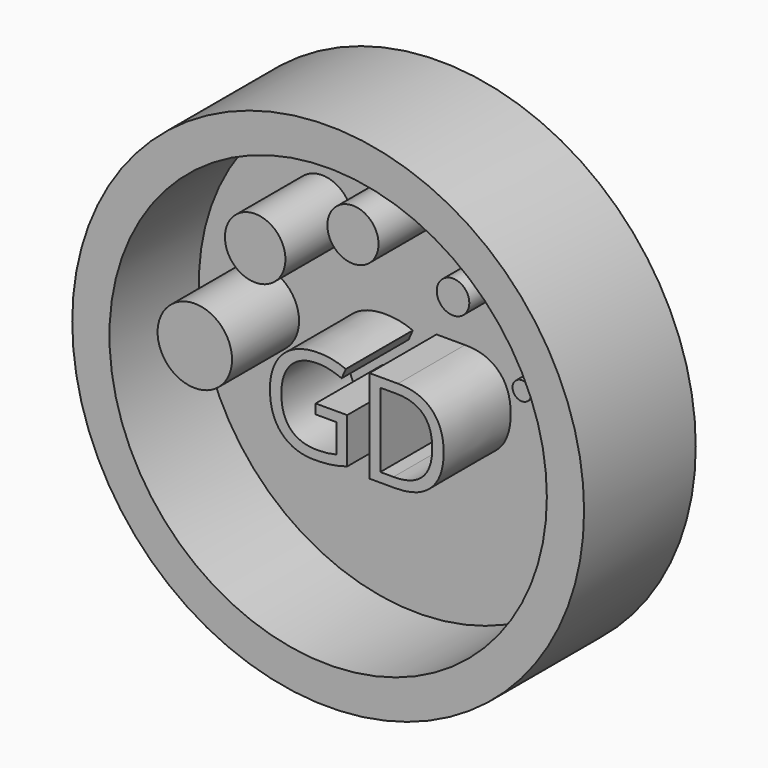
from build123d import *

# Parameters (mm, degrees)
F0_R         = 27.5
F0_R_2       = 23.5
F1_DEPTH     = 12
F2_R         = 27.5
F3_DEPTH     = 3
F4_R         = 4
F4_R_2       = 3.25
F4_R_3       = 2.75
F4_R_4       = 1.75
F4_R_5       = 1
F5_DEPTH     = 9
F6_TEXT_SIZE = 13.9870023362
F7_DEPTH     = 9


# Not quite as in the source:
# - Text() gives the source's letters only with a copy of the font that has no kerning and outlines rounded to 1/6400 em; it was checked with that copy


with BuildPart() as f1:
    # F0 (on Front) → F1 (new body)
    with BuildSketch(Plane.XZ):
        Circle(F0_R)
        Circle(F0_R_2, mode=Mode.SUBTRACT)
    extrude(amount=F1_DEPTH)

    # F2 (on Front) → F3 (join)
    with BuildSketch(Plane.XZ):
        Circle(F2_R)
    extrude(amount=-F3_DEPTH)

    # F4 (on Front) → F5 (join)
    with BuildSketch(Plane.XZ):
        with Locations((-16.7306032029, 0)):
            Circle(F4_R)
        with Locations((-10.2427472395, 11.3465488841)):
            Circle(F4_R_2)
        with Locations((0.264364346, 16.0439414204)):
            Circle(F4_R_3)
        with Locations((11.017489247, 13.6466622353)):
            Circle(F4_R_4)
        with Locations((18.4116128074, 7.1751135777)):
            Circle(F4_R_5)
    extrude(amount=F5_DEPTH)

    # F6 (on Front) → F7 (join)
    with BuildSketch(Plane.XZ):
        with Locations((-9.5128534346, -6.4618588295)):
            Text('GD', F6_TEXT_SIZE, font='Open Sans', text_align=(TextAlign.LEFT, TextAlign.BOTTOM))
    extrude(amount=F7_DEPTH)


solid = f1.part
